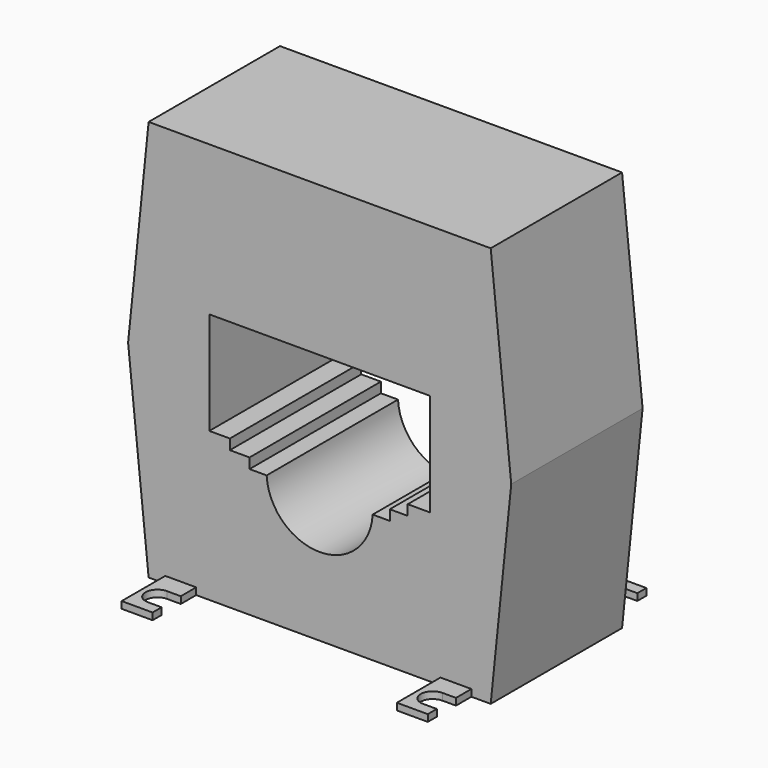
from build123d import *

# Parameters (mm, degrees)
F1_DEPTH = 24
F3_DEPTH = 2
F4_DEPTH = 24
F5_DEPTH = 5


# Not quite as in the source:
# - a feature names something its author has since deleted; it is built from what else it names


with BuildPart() as f1:
    # F0 (on Front) → F1 (new body, symmetric)
    with BuildSketch(Plane.XZ):
        Polygon((-40, -58.5), (0, -58.5), (40, -58.5), (50, -58.5), (56, 0), (50, 58.75), (0, 58.75), (-50, 58.75), (-56, 0), (-50, -58.5), align=None)
        with BuildLine():
            Line((-32.25, 15), (0, 15))
            Line((0, 15), (32.25, 15))
            Line((32.25, 15), (32.25, -15))
            Line((32.25, -15), (25.75, -15))
            Line((25.75, -15), (25.75, -18))
            Line((25.75, -18), (20.5, -18))
            Line((20.5, -18), (20.5, -21))
            Line((20.5, -21), (15.5, -21))
            ThreePointArc((15.5, -21), (0, -35.6865517328), (-15.5, -21))
            Line((-15.5, -21), (-20.5, -21))
            Line((-20.5, -21), (-20.5, -18))
            Line((-20.5, -18), (-26.25, -18))
            Line((-26.25, -18), (-26.25, -15))
            Line((-26.25, -15), (-32.25, -15))
            Line((-32.25, -15), (-32.25, 15))
        make_face(mode=Mode.SUBTRACT)
    extrude(amount=F1_DEPTH, both=True)

    # F0 (on Front) → F4 (cut, symmetric)
    with BuildSketch(Plane.XZ):
        with BuildLine():
            Line((32.25, 15), (0, 15))
            Line((0, 15), (-32.25, 15))
            Line((-32.25, 15), (-32.25, -15))
            Line((-32.25, -15), (-26.25, -15))
            Line((-26.25, -15), (-26.25, -18))
            Line((-26.25, -18), (-20.5, -18))
            Line((-20.5, -18), (-20.5, -21))
            Line((-20.5, -21), (-15.5, -21))
            ThreePointArc((-15.5, -21), (0, -35.6865517328), (15.5, -21))
            Line((15.5, -21), (20.5, -21))
            Line((20.5, -21), (20.5, -18))
            Line((20.5, -18), (25.75, -18))
            Line((25.75, -18), (25.75, -15))
            Line((25.75, -15), (32.25, -15))
            Line((32.25, -15), (32.25, 15))
        make_face()
    extrude(amount=F4_DEPTH, both=True, mode=Mode.SUBTRACT)

    # F2 (on face) → F5 (cut)
    with BuildSketch(Plane(origin=(0, 0, -58.5), x_dir=(1, 0, 0), z_dir=(0, 0, -1))):
        with BuildLine():
            Line((-40.0934517384, -33.1348065302), (-40.0934517384, -29.6348065302))
            ThreePointArc((-40.0934517384, -29.6348065302), (-43.5934517384, -33.1348065302), (-40.0934517384, -36.6348065302))
            Line((-40.0934517384, -36.6348065302), (-40.0934517384, -33.1348065302))
        make_face()
        with BuildLine():
            ThreePointArc((-36.5934517384, -33.1348065302), (-37.6185780042, -30.659932796), (-40.0934517384, -29.6348065302))
            Line((-40.0934517384, -29.6348065302), (-40.0934517384, -33.1348065302))
            Line((-40.0934517384, -33.1348065302), (-40.0934517384, -36.6348065302))
            ThreePointArc((-40.0934517384, -36.6348065302), (-37.6185780042, -35.6096802643), (-36.5934517384, -33.1348065302))
        make_face()
        with BuildLine():
            Line((-36.0934517384, -36.6348065302), (-36.0934517384, -29.6348065302))
            Line((-36.0934517384, -29.6348065302), (-40.0934517384, -29.6348065302))
            ThreePointArc((-40.0934517384, -29.6348065302), (-37.6185780042, -30.659932796), (-36.5934517384, -33.1348065302))
            ThreePointArc((-36.5934517384, -33.1348065302), (-37.6185780042, -35.6096802643), (-40.0934517384, -36.6348065302))
            Line((-40.0934517384, -36.6348065302), (-36.0934517384, -36.6348065302))
        make_face()
        with BuildLine():
            ThreePointArc((-40.0934517384, 36.6348065302), (-43.5934517384, 33.1348065302), (-40.0934517384, 29.6348065302))
            Line((-40.0934517384, 29.6348065302), (-40.0934517384, 33.1348065302))
            Line((-40.0934517384, 33.1348065302), (-40.0934517384, 36.6348065302))
        make_face()
        with BuildLine():
            Line((-40.0934517384, 33.1348065302), (-40.0934517384, 29.6348065302))
            ThreePointArc((-40.0934517384, 29.6348065302), (-37.6185780042, 30.659932796), (-36.5934517384, 33.1348065302))
            ThreePointArc((-36.5934517384, 33.1348065302), (-37.6185780042, 35.6096802643), (-40.0934517384, 36.6348065302))
            Line((-40.0934517384, 36.6348065302), (-40.0934517384, 33.1348065302))
        make_face()
        with BuildLine():
            Line((-40.0934517384, 29.6348065302), (-36.0934517384, 29.6348065302))
            Line((-36.0934517384, 29.6348065302), (-36.0934517384, 36.6348065302))
            Line((-36.0934517384, 36.6348065302), (-40.0934517384, 36.6348065302))
            ThreePointArc((-40.0934517384, 36.6348065302), (-37.6185780042, 35.6096802643), (-36.5934517384, 33.1348065302))
            ThreePointArc((-36.5934517384, 33.1348065302), (-37.6185780042, 30.659932796), (-40.0934517384, 29.6348065302))
        make_face()
        with BuildLine():
            Line((40.3557159007, -36.6348065302), (44.3557159007, -36.6348065302))
            Line((44.3557159007, -36.6348065302), (44.3557159007, -29.6348065302))
            Line((44.3557159007, -29.6348065302), (40.3557159007, -29.6348065302))
            ThreePointArc((40.3557159007, -29.6348065302), (42.8305896348, -30.659932796), (43.8557159007, -33.1348065302))
            ThreePointArc((43.8557159007, -33.1348065302), (42.8305896348, -35.6096802643), (40.3557159007, -36.6348065302))
        make_face()
        with BuildLine():
            Line((40.3557159007, -33.1348065302), (40.3557159007, -36.6348065302))
            ThreePointArc((40.3557159007, -36.6348065302), (42.8305896348, -35.6096802643), (43.8557159007, -33.1348065302))
            ThreePointArc((43.8557159007, -33.1348065302), (42.8305896348, -30.659932796), (40.3557159007, -29.6348065302))
            Line((40.3557159007, -29.6348065302), (40.3557159007, -33.1348065302))
        make_face()
        with BuildLine():
            ThreePointArc((40.3557159007, -29.6348065302), (36.8557159007, -33.1348065302), (40.3557159007, -36.6348065302))
            Line((40.3557159007, -36.6348065302), (40.3557159007, -33.1348065302))
            Line((40.3557159007, -33.1348065302), (40.3557159007, -29.6348065302))
        make_face()
        with BuildLine():
            ThreePointArc((40.3557159007, 36.6348065302), (36.8557159007, 33.1348065302), (40.3557159007, 29.6348065302))
            Line((40.3557159007, 29.6348065302), (40.3557159007, 33.1348065302))
            Line((40.3557159007, 33.1348065302), (40.3557159007, 36.6348065302))
        make_face()
        with BuildLine():
            Line((40.3557159007, 33.1348065302), (40.3557159007, 29.6348065302))
            ThreePointArc((40.3557159007, 29.6348065302), (42.8305896348, 30.659932796), (43.8557159007, 33.1348065302))
            ThreePointArc((43.8557159007, 33.1348065302), (42.8305896348, 35.6096802643), (40.3557159007, 36.6348065302))
            Line((40.3557159007, 36.6348065302), (40.3557159007, 33.1348065302))
        make_face()
        with BuildLine():
            Line((40.3557159007, 29.6348065302), (44.3557159007, 29.6348065302))
            Line((44.3557159007, 29.6348065302), (44.3557159007, 36.6348065302))
            Line((44.3557159007, 36.6348065302), (40.3557159007, 36.6348065302))
            ThreePointArc((40.3557159007, 36.6348065302), (42.8305896348, 35.6096802643), (43.8557159007, 33.1348065302))
            ThreePointArc((43.8557159007, 33.1348065302), (42.8305896348, 30.659932796), (40.3557159007, 29.6348065302))
        make_face()
    extrude(amount=-F5_DEPTH, mode=Mode.SUBTRACT)


with BuildPart() as f3:
    # F2 (on face) → F3 (new body)
    with BuildSketch(Plane(origin=(0, 0, -58.5), x_dir=(1, 0, 0), z_dir=(0, 0, -1))):
        with BuildLine():
            Line((-45.1397926509, 39.9301091), (-45.1397926509, 24))
            Line((-45.1397926509, 24), (-36.0934517384, 24))
            Line((-36.0934517384, 24), (-36.0934517384, 29.6348065302))
            Line((-36.0934517384, 29.6348065302), (-40.0934517384, 29.6348065302))
            ThreePointArc((-40.0934517384, 29.6348065302), (-43.5934517384, 33.1348065302), (-40.0934517384, 36.6348065302))
            Line((-40.0934517384, 36.6348065302), (-36.0934517384, 36.6348065302))
            Line((-36.0934517384, 36.6348065302), (-36.0934517384, 39.9301091))
            Line((-36.0934517384, 39.9301091), (-45.1397926509, 39.9301091))
        make_face()
    extrude(amount=-F3_DEPTH)


with BuildPart() as f3b:
    # F2 (on face) → F3, piece 2 (new body)
    with BuildSketch(Plane(origin=(0, 0, -58.5), x_dir=(1, 0, 0), z_dir=(0, 0, -1))):
        with BuildLine():
            Line((35.3093749881, -39.9301091), (44.3557159007, -39.9301091))
            Line((44.3557159007, -39.9301091), (44.3557159007, -36.6348065302))
            Line((44.3557159007, -36.6348065302), (40.3557159007, -36.6348065302))
            ThreePointArc((40.3557159007, -36.6348065302), (36.8557159007, -33.1348065302), (40.3557159007, -29.6348065302))
            Line((40.3557159007, -29.6348065302), (44.3557159007, -29.6348065302))
            Line((44.3557159007, -29.6348065302), (44.3557159007, -24))
            Line((44.3557159007, -24), (35.3093749881, -24))
            Line((35.3093749881, -24), (35.3093749881, -39.9301091))
        make_face()
    extrude(amount=-F3_DEPTH)


with BuildPart() as f3c:
    # F2 (on face) → F3, piece 3 (new body)
    with BuildSketch(Plane(origin=(0, 0, -58.5), x_dir=(1, 0, 0), z_dir=(0, 0, -1))):
        with BuildLine():
            Line((-36.0934517384, -29.6348065302), (-36.0934517384, -24))
            Line((-36.0934517384, -24), (-45.1397926509, -24))
            Line((-45.1397926509, -24), (-45.1397926509, -39.9301091))
            Line((-45.1397926509, -39.9301091), (-36.0934517384, -39.9301091))
            Line((-36.0934517384, -39.9301091), (-36.0934517384, -36.6348065302))
            Line((-36.0934517384, -36.6348065302), (-40.0934517384, -36.6348065302))
            ThreePointArc((-40.0934517384, -36.6348065302), (-43.5934517384, -33.1348065302), (-40.0934517384, -29.6348065302))
            Line((-40.0934517384, -29.6348065302), (-36.0934517384, -29.6348065302))
        make_face()
    extrude(amount=-F3_DEPTH)


with BuildPart() as f3d:
    # F2 (on face) → F3, piece 4 (new body)
    with BuildSketch(Plane(origin=(0, 0, -58.5), x_dir=(1, 0, 0), z_dir=(0, 0, -1))):
        with BuildLine():
            Line((35.3093749881, 24), (44.3557159007, 24))
            Line((44.3557159007, 24), (44.3557159007, 29.6348065302))
            Line((44.3557159007, 29.6348065302), (40.3557159007, 29.6348065302))
            ThreePointArc((40.3557159007, 29.6348065302), (36.8557159007, 33.1348065302), (40.3557159007, 36.6348065302))
            Line((40.3557159007, 36.6348065302), (44.3557159007, 36.6348065302))
            Line((44.3557159007, 36.6348065302), (44.3557159007, 39.9301091))
            Line((44.3557159007, 39.9301091), (35.3093749881, 39.9301091))
            Line((35.3093749881, 39.9301091), (35.3093749881, 24))
        make_face()
    extrude(amount=-F3_DEPTH)


solid = Compound([f1.part, f3.part, f3b.part, f3c.part, f3d.part])
